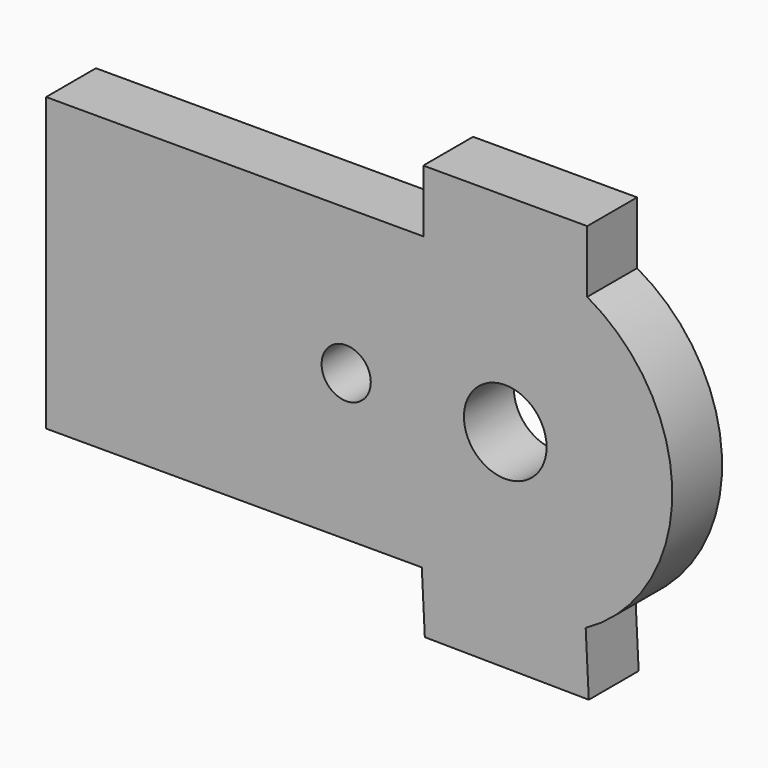
from build123d import *

# Parameters (mm, degrees)
F0_R     = 1.905
F0_R_2   = 3.2
F1_DEPTH = 4.826


# Not quite as in the source:
# - a feature names something its author has since deleted; it is built from what else it names


with BuildPart() as f1:
    # F0 (on Front) → F1 (new body)
    with BuildSketch(Plane.XZ):
        with BuildLine():
            Line((-6.2288098753, -16.020498732), (6.4704601492, -16.156663498))
            Line((6.4704601492, -16.156663498), (6.2288098753, -11.3367173214))
            ThreePointArc((6.2288098753, -11.3367173214), (12.9350076718, -0.0693442092), (6.35, 11.2692826786))
            Line((6.35, 11.2692826786), (6.35, 16.0952826786))
            Line((6.35, 16.0952826786), (-6.35, 16.0952826786))
            Line((-6.35, 16.0952826786), (-6.35, 11.2692826786))
            Line((-6.35, 11.2692826786), (-35.56, 11.2692826786))
            Line((-35.56, 11.2692826786), (-35.56, -11.3367173214))
            Line((-35.56, -11.3367173214), (-6.4636334645, -11.3367173214))
            Line((-6.4636334645, -11.3367173214), (-6.2288098753, -16.020498732))
        make_face()
        with Locations((-12.319, 0)):
            Circle(F0_R, mode=Mode.SUBTRACT)
        Circle(F0_R_2, mode=Mode.SUBTRACT)
    extrude(amount=F1_DEPTH)


solid = f1.part
